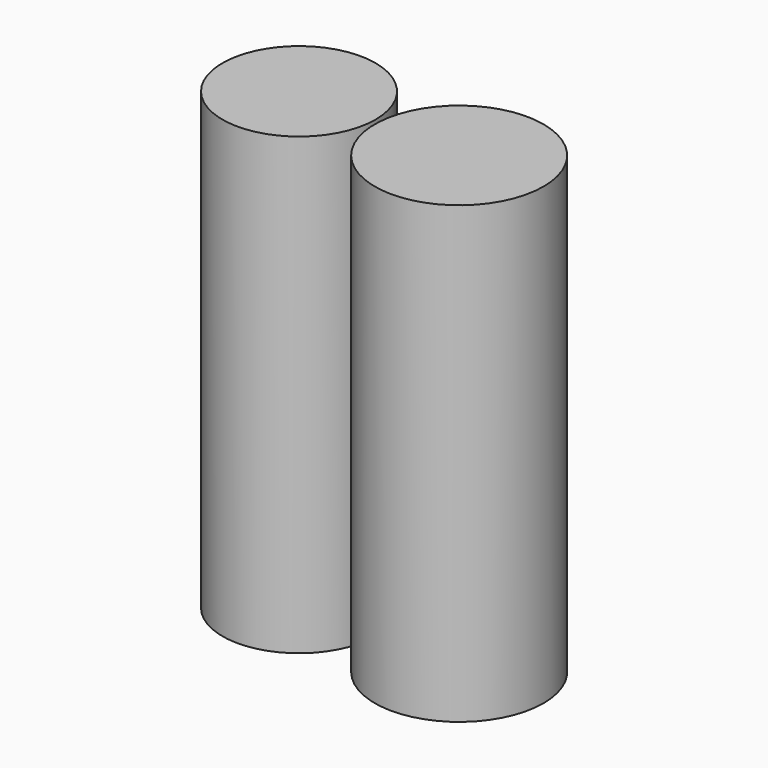
from build123d import *

# Parameters (mm, degrees)
F0_R     = 21.3736978342
F1_DEPTH = 127
F0_R_2   = 23.5556539699


# Not quite as in the source:
# - the program builds the solid bodies; features that only make, move or delete a surface that nothing else refers to are left out


with BuildPart() as f1:
    # F0 (on Top) → F1 (new body)
    with BuildSketch(Plane.XY):
        with Locations((-36.1441485584, 27.2724032402)):
            Circle(F0_R)
    extrude(amount=F1_DEPTH)


with BuildPart() as f1b:
    # F0 (on Top) → F1, piece 2 (new body)
    with BuildSketch(Plane.XY):
        with Locations((10.0217889994, 25.4651959985)):
            Circle(F0_R_2)
    extrude(amount=F1_DEPTH)


solid = Compound([f1.part, f1b.part])
